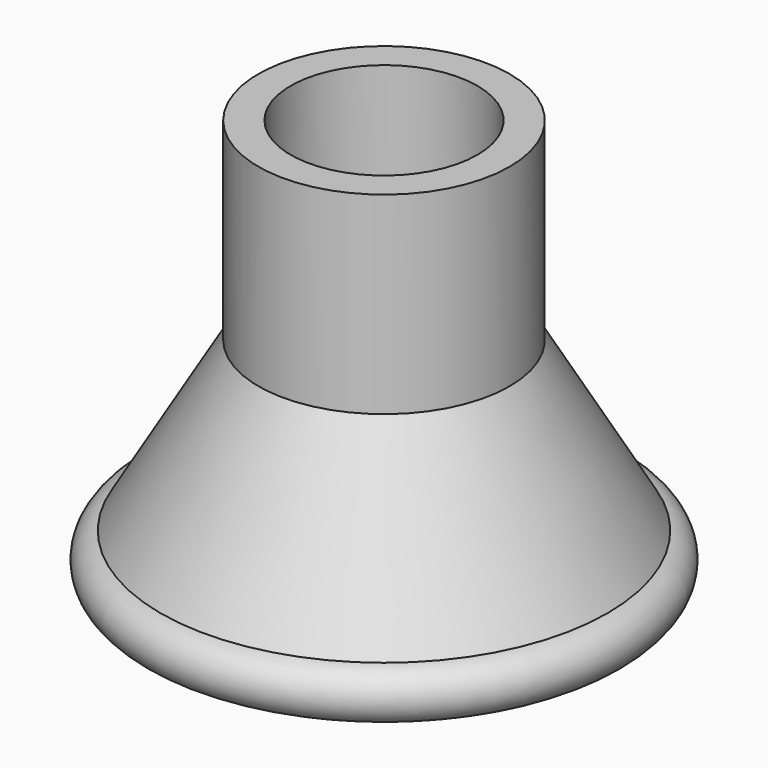
from build123d import *


# Not quite as in the source:
# - a feature names something its author has since deleted; it is built from what else it names


with BuildPart() as f1:
    # F0 (on Front) → F1 (revolve)
    with BuildSketch(Plane.XZ):
        with BuildLine():
            Line((9.2075, 19.05), (9.2075, 2.54))
            Line((9.2075, 2.54), (7.9375, 2.54))
            Line((7.9375, 2.54), (7.9375, 0))
            Line((7.9375, 0), (19.05, -19.05))
            ThreePointArc((19.05, -19.05), (23.2206068806, -20.9974910015), (22.0363946464, -16.5495336796))
            Line((22.0363946464, -16.5495336796), (12.3825, 0))
            Line((12.3825, 0), (12.3825, 19.05))
            Line((12.3825, 19.05), (9.2075, 19.05))
        make_face()
    revolve(axis=Axis((0, 0, -5.8383159339), (0, 0, -1)))


solid = f1.part
